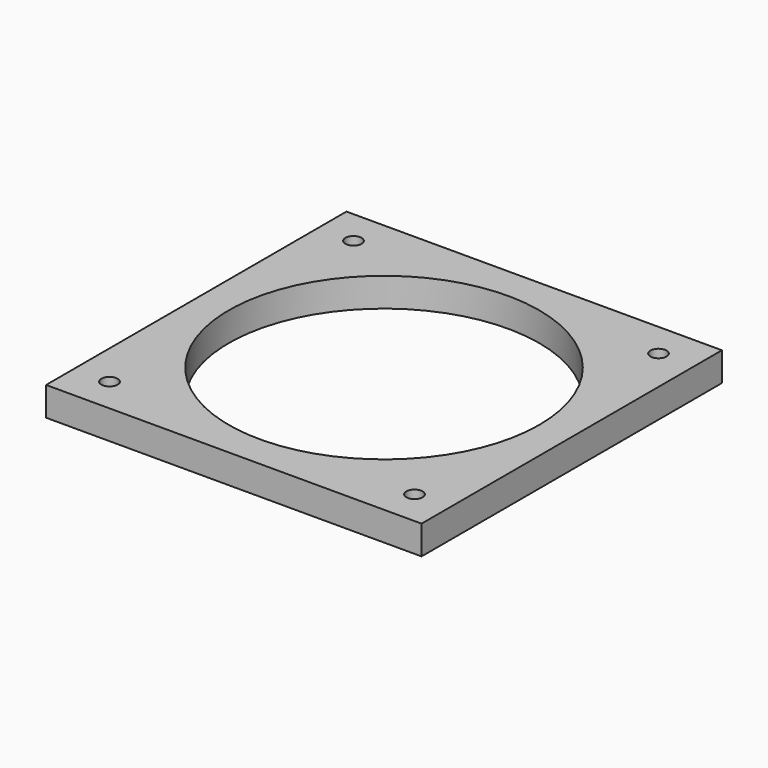
from build123d import *

# Parameters (mm, degrees)
F0_W     = 82.55
F0_H     = 82.55
F0_R     = 1.778
F0_R_2   = 34.13125
F1_DEPTH = 6.35


# Not quite as in the source:
# - a length typed as a fraction of an inch, garbled in the dataset ("3 / 203.2 mm" for 3/8 in), is restored


with BuildPart() as f1:
    # F0 (on Top) → F1 (new body)
    with BuildSketch(Plane.XY):
        Rectangle(F0_W, F0_H)
        with Locations((-33.528, -33.528)):
            Circle(F0_R, mode=Mode.SUBTRACT)
        with Locations((33.528, -33.528)):
            Circle(F0_R, mode=Mode.SUBTRACT)
        with Locations((-33.528, 33.528)):
            Circle(F0_R, mode=Mode.SUBTRACT)
        Circle(F0_R_2, mode=Mode.SUBTRACT)
        with Locations((33.528, 33.528)):
            Circle(F0_R, mode=Mode.SUBTRACT)
    extrude(amount=F1_DEPTH)


solid = f1.part
